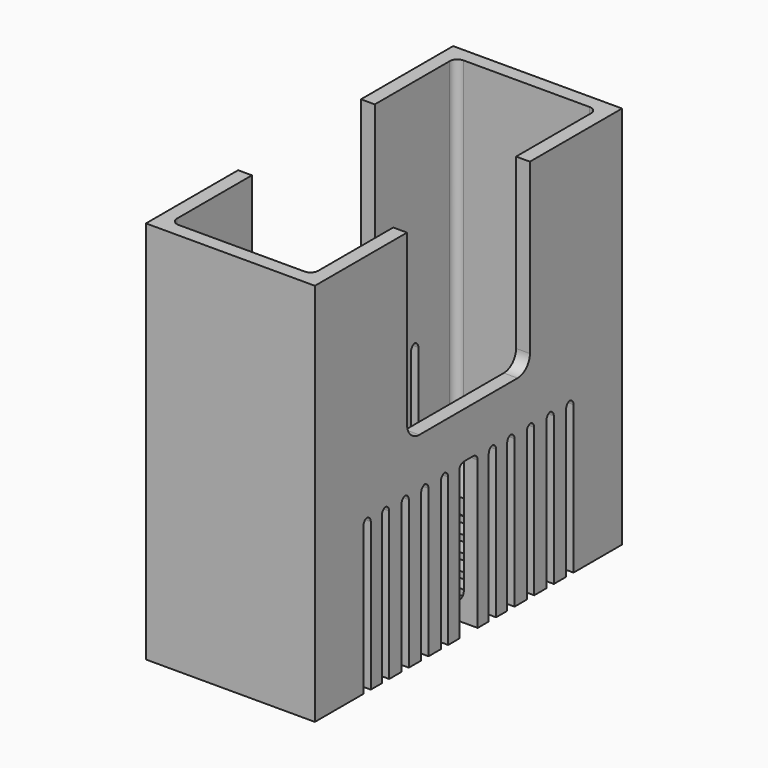
from build123d import *

# Parameters (mm, degrees)
F0_W            = 22
F0_H            = 50
F1_DEPTH        = 50
F2_T            = -1.8
F3_R            = 2
F4_W            = 33.5534993559
F4_H            = 3
F4_W_2          = 30.2066039294
F4_H_2          = 1.2
F4_W_3          = 26.0875225067
F4_W_4          = 25.4990821704
F4_W_5          = 26.8721096218
F4_W_6          = 25.5971541628
F4_W_7          = 23.243393749
F4_W_8          = 31.1466334388
F4_W_9          = 36.8653591722
F4_W_10         = 30.2834836766
F4_W_11         = 31.6123114899
F5_DEPTH        = 20
F6_W            = 20.4323772341
F6_H            = 6
F7_DEPTH        = 2
F8_W            = 20.5352026969
F8_H            = 6
F9_DEPTH        = 2
F10_R           = 1
F12_D           = 3.4
F12_CSINK_D     = 6.72
F12_CSINK_ANGLE = 90
F13_T1_DEPTH    = 1.8
F13_T3_DEPTH    = 1.8
F15_DEPTH       = 22.001


# Not quite as in the source:
# - a fillet or chamfer that OpenCascade refuses, or shapes differently, is made with other operations: its cross-section is extruded or revolved along the edge and cut away or added


with BuildPart() as f1:
    # F0 (on Top) → F1 (new body)
    with BuildSketch(Plane.XY):
        Rectangle(F0_W, F0_H)
    extrude(amount=F1_DEPTH)

    # F2
    f2_openings = [f1.faces().sort_by_distance(p)[0] for p in [
        (0, 0, 50),
    ]]
    offset(amount=F2_T, openings=f2_openings)

    # F3
    f3_edges = [f1.edges().sort_by_distance(p)[0] for p in [
        (9.2, 0, 1.8),
        (-9.2, 0, 1.8),
    ]]
    fillet(f3_edges, radius=F3_R)

    # F4 (on face) → F5 (cut)
    with BuildSketch(Plane(origin=(0, 0, 0), x_dir=(1, 0, 0), z_dir=(0, 0, -1))):
        with Locations((0.5022748373, 0)):
            Rectangle(F4_W, F4_H)
        with Locations((0.0301385298, 3.9)):
            Rectangle(F4_W_2, F4_H_2)
        with Locations((-0.4602279514, 10.3)):
            Rectangle(F4_W_3, F4_H_2)
        with Locations((-1.1467416771, -6.9)):
            Rectangle(F4_W_4, F4_H_2)
        with Locations((-0.6563747302, -10.1)):
            Rectangle(F4_W_5, F4_H_2)
        with Locations((-0.6073382683, -3.9)):
            Rectangle(F4_W_6, F4_H_2)
        with Locations((-0.2150442451, 7.1)):
            Rectangle(F4_W_7, F4_H_2)
        with Locations((0.075826887, 13.5)):
            Rectangle(F4_W_8, F4_H_2)
        with Locations((0.9949086234, -13.3)):
            Rectangle(F4_W_9, F4_H_2)
        with Locations((0.5074017681, 16.5)):
            Rectangle(F4_W_10, F4_H_2)
        with Locations((1.4125197195, -16.5)):
            Rectangle(F4_W_11, F4_H_2)
    extrude(amount=-F5_DEPTH, mode=Mode.SUBTRACT)

    # F6 (on face) → F7 (join)
    with BuildSketch(Plane.XY.offset(1.8)):
        with Locations((0.1267548651, 20.2)):
            Rectangle(F6_W, F6_H)
    extrude(amount=F7_DEPTH)

    # F8 (on face) → F9 (join)
    with BuildSketch(Plane.XY.offset(1.8)):
        with Locations((-0.0829612836, -20.2)):
            Rectangle(F8_W, F8_H)
    extrude(amount=F9_DEPTH)

    # F10
    f10_edges = [f1.edges().sort_by_distance(p)[0] for p in [
        (-9.2, -23.2, 26.9),
        (9.2, -23.2, 26.9),
        (9.2, 23.2, 26.9),
        (-9.2, 23.2, 26.9),
    ]]
    fillet(f10_edges, radius=F10_R)

    # F12 (through all)
    with Locations(Plane(origin=(0, 0, 0), x_dir=(1, 0, 0), z_dir=(0, 0, -1))):
        with Locations((0, 21), (0, -21)):
            CounterSinkHole(F12_D / 2, F12_CSINK_D / 2, counter_sink_angle=F12_CSINK_ANGLE)

    # F13: fillet of radius 0.75 on 44 edges, made by hand

    # F13_s2 → F13_t1 (join)
    with BuildSketch(Plane.YZ.offset(-11)):
        with BuildLine():
            ThreePointArc((-1.5, 19.25), (-1.2803300859, 19.7803300859), (-0.75, 20))
            Line((-0.75, 20), (-1.5, 20))
            Line((-1.5, 20), (-1.5, 19.25))
        make_face()
        with BuildLine():
            ThreePointArc((1.5, 19.25), (1.2803300859, 19.7803300859), (0.75, 20))
            Line((0.75, 20), (1.5, 20))
            Line((1.5, 20), (1.5, 19.25))
        make_face()
        with BuildLine():
            ThreePointArc((13.9, 19.25), (13.6803300859, 19.7803300859), (13.15, 20))
            Line((13.15, 20), (13.9, 20))
            Line((13.9, 20), (13.9, 19.25))
        make_face()
        with BuildLine():
            ThreePointArc((12.7, 19.25), (12.9196699141, 19.7803300859), (13.45, 20))
            Line((13.45, 20), (12.7, 20))
            Line((12.7, 20), (12.7, 19.25))
        make_face()
        with BuildLine():
            ThreePointArc((10.7, 19.25), (10.4803300859, 19.7803300859), (9.95, 20))
            Line((9.95, 20), (10.7, 20))
            Line((10.7, 20), (10.7, 19.25))
        make_face()
        with BuildLine():
            ThreePointArc((9.5, 19.25), (9.7196699141, 19.7803300859), (10.25, 20))
            Line((10.25, 20), (9.5, 20))
            Line((9.5, 20), (9.5, 19.25))
        make_face()
        with BuildLine():
            ThreePointArc((7.5, 19.25), (7.2803300859, 19.7803300859), (6.75, 20))
            Line((6.75, 20), (7.5, 20))
            Line((7.5, 20), (7.5, 19.25))
        make_face()
        with BuildLine():
            ThreePointArc((6.3, 19.25), (6.5196699141, 19.7803300859), (7.05, 20))
            Line((7.05, 20), (6.3, 20))
            Line((6.3, 20), (6.3, 19.25))
        make_face()
        with BuildLine():
            ThreePointArc((4.5, 19.25), (4.2803300859, 19.7803300859), (3.75, 20))
            Line((3.75, 20), (4.5, 20))
            Line((4.5, 20), (4.5, 19.25))
        make_face()
        with BuildLine():
            ThreePointArc((3.3, 19.25), (3.5196699141, 19.7803300859), (4.05, 20))
            Line((4.05, 20), (3.3, 20))
            Line((3.3, 20), (3.3, 19.25))
        make_face()
        with BuildLine():
            ThreePointArc((-3.3, 19.25), (-3.5196699141, 19.7803300859), (-4.05, 20))
            Line((-4.05, 20), (-3.3, 20))
            Line((-3.3, 20), (-3.3, 19.25))
        make_face()
        with BuildLine():
            ThreePointArc((-6.5, 19.25), (-6.7196699141, 19.7803300859), (-7.25, 20))
            Line((-7.25, 20), (-6.5, 20))
            Line((-6.5, 20), (-6.5, 19.25))
        make_face()
        with BuildLine():
            ThreePointArc((-9.7, 19.25), (-9.9196699141, 19.7803300859), (-10.45, 20))
            Line((-10.45, 20), (-9.7, 20))
            Line((-9.7, 20), (-9.7, 19.25))
        make_face()
        with BuildLine():
            ThreePointArc((-12.9, 19.25), (-13.1196699141, 19.7803300859), (-13.65, 20))
            Line((-13.65, 20), (-12.9, 20))
            Line((-12.9, 20), (-12.9, 19.25))
        make_face()
        with BuildLine():
            ThreePointArc((-14.1, 19.25), (-13.8803300859, 19.7803300859), (-13.35, 20))
            Line((-13.35, 20), (-14.1, 20))
            Line((-14.1, 20), (-14.1, 19.25))
        make_face()
        with BuildLine():
            ThreePointArc((-10.9, 19.25), (-10.6803300859, 19.7803300859), (-10.15, 20))
            Line((-10.15, 20), (-10.9, 20))
            Line((-10.9, 20), (-10.9, 19.25))
        make_face()
        with BuildLine():
            ThreePointArc((-7.7, 19.25), (-7.4803300859, 19.7803300859), (-6.95, 20))
            Line((-6.95, 20), (-7.7, 20))
            Line((-7.7, 20), (-7.7, 19.25))
        make_face()
        with BuildLine():
            ThreePointArc((-4.5, 19.25), (-4.2803300859, 19.7803300859), (-3.75, 20))
            Line((-3.75, 20), (-4.5, 20))
            Line((-4.5, 20), (-4.5, 19.25))
        make_face()
        with BuildLine():
            ThreePointArc((15.9, 19.25), (16.1196699141, 19.7803300859), (16.65, 20))
            Line((16.65, 20), (15.9, 20))
            Line((15.9, 20), (15.9, 19.25))
        make_face()
        with BuildLine():
            ThreePointArc((17.1, 19.25), (16.8803300859, 19.7803300859), (16.35, 20))
            Line((16.35, 20), (17.1, 20))
            Line((17.1, 20), (17.1, 19.25))
        make_face()
        with BuildLine():
            ThreePointArc((-17.1, 19.25), (-16.8803300859, 19.7803300859), (-16.35, 20))
            Line((-16.35, 20), (-17.1, 20))
            Line((-17.1, 20), (-17.1, 19.25))
        make_face()
        with BuildLine():
            ThreePointArc((-15.9, 19.25), (-16.1196699141, 19.7803300859), (-16.65, 20))
            Line((-16.65, 20), (-15.9, 20))
            Line((-15.9, 20), (-15.9, 19.25))
        make_face()
    extrude(amount=F13_T1_DEPTH)

    # F13_s4 → F13_t3 (join)
    with BuildSketch(Plane.YZ.offset(9.2)):
        with BuildLine():
            ThreePointArc((1.5, 19.25), (1.2803300859, 19.7803300859), (0.75, 20))
            Line((0.75, 20), (1.5, 20))
            Line((1.5, 20), (1.5, 19.25))
        make_face()
        with BuildLine():
            ThreePointArc((-1.5, 19.25), (-1.2803300859, 19.7803300859), (-0.75, 20))
            Line((-0.75, 20), (-1.5, 20))
            Line((-1.5, 20), (-1.5, 19.25))
        make_face()
        with BuildLine():
            ThreePointArc((-13.65, 20), (-13.1196699141, 19.7803300859), (-12.9, 19.25))
            Line((-12.9, 19.25), (-12.9, 20))
            Line((-12.9, 20), (-13.65, 20))
        make_face()
        with BuildLine():
            ThreePointArc((-10.45, 20), (-9.9196699141, 19.7803300859), (-9.7, 19.25))
            Line((-9.7, 19.25), (-9.7, 20))
            Line((-9.7, 20), (-10.45, 20))
        make_face()
        with BuildLine():
            ThreePointArc((-7.25, 20), (-6.7196699141, 19.7803300859), (-6.5, 19.25))
            Line((-6.5, 19.25), (-6.5, 20))
            Line((-6.5, 20), (-7.25, 20))
        make_face()
        with BuildLine():
            ThreePointArc((-4.05, 20), (-3.5196699141, 19.7803300859), (-3.3, 19.25))
            Line((-3.3, 19.25), (-3.3, 20))
            Line((-3.3, 20), (-4.05, 20))
        make_face()
        with BuildLine():
            ThreePointArc((4.5, 19.25), (4.2803300859, 19.7803300859), (3.75, 20))
            Line((3.75, 20), (4.5, 20))
            Line((4.5, 20), (4.5, 19.25))
        make_face()
        with BuildLine():
            ThreePointArc((7.5, 19.25), (7.2803300859, 19.7803300859), (6.75, 20))
            Line((6.75, 20), (7.5, 20))
            Line((7.5, 20), (7.5, 19.25))
        make_face()
        with BuildLine():
            ThreePointArc((10.7, 19.25), (10.4803300859, 19.7803300859), (9.95, 20))
            Line((9.95, 20), (10.7, 20))
            Line((10.7, 20), (10.7, 19.25))
        make_face()
        with BuildLine():
            ThreePointArc((13.9, 19.25), (13.6803300859, 19.7803300859), (13.15, 20))
            Line((13.15, 20), (13.9, 20))
            Line((13.9, 20), (13.9, 19.25))
        make_face()
        with BuildLine():
            ThreePointArc((-14.1, 19.25), (-13.8803300859, 19.7803300859), (-13.35, 20))
            Line((-13.35, 20), (-14.1, 20))
            Line((-14.1, 20), (-14.1, 19.25))
        make_face()
        with BuildLine():
            ThreePointArc((-10.9, 19.25), (-10.6803300859, 19.7803300859), (-10.15, 20))
            Line((-10.15, 20), (-10.9, 20))
            Line((-10.9, 20), (-10.9, 19.25))
        make_face()
        with BuildLine():
            ThreePointArc((-7.7, 19.25), (-7.4803300859, 19.7803300859), (-6.95, 20))
            Line((-6.95, 20), (-7.7, 20))
            Line((-7.7, 20), (-7.7, 19.25))
        make_face()
        with BuildLine():
            ThreePointArc((-4.5, 19.25), (-4.2803300859, 19.7803300859), (-3.75, 20))
            Line((-3.75, 20), (-4.5, 20))
            Line((-4.5, 20), (-4.5, 19.25))
        make_face()
        with BuildLine():
            ThreePointArc((4.05, 20), (3.5196699141, 19.7803300859), (3.3, 19.25))
            Line((3.3, 19.25), (3.3, 20))
            Line((3.3, 20), (4.05, 20))
        make_face()
        with BuildLine():
            ThreePointArc((7.05, 20), (6.5196699141, 19.7803300859), (6.3, 19.25))
            Line((6.3, 19.25), (6.3, 20))
            Line((6.3, 20), (7.05, 20))
        make_face()
        with BuildLine():
            ThreePointArc((10.25, 20), (9.7196699141, 19.7803300859), (9.5, 19.25))
            Line((9.5, 19.25), (9.5, 20))
            Line((9.5, 20), (10.25, 20))
        make_face()
        with BuildLine():
            ThreePointArc((13.45, 20), (12.9196699141, 19.7803300859), (12.7, 19.25))
            Line((12.7, 19.25), (12.7, 20))
            Line((12.7, 20), (13.45, 20))
        make_face()
        with BuildLine():
            ThreePointArc((-17.1, 19.25), (-16.8803300859, 19.7803300859), (-16.35, 20))
            Line((-16.35, 20), (-17.1, 20))
            Line((-17.1, 20), (-17.1, 19.25))
        make_face()
        with BuildLine():
            ThreePointArc((-16.65, 20), (-16.1196699141, 19.7803300859), (-15.9, 19.25))
            Line((-15.9, 19.25), (-15.9, 20))
            Line((-15.9, 20), (-16.65, 20))
        make_face()
        with BuildLine():
            ThreePointArc((17.1, 19.25), (16.8803300859, 19.7803300859), (16.35, 20))
            Line((16.35, 20), (17.1, 20))
            Line((17.1, 20), (17.1, 19.25))
        make_face()
        with BuildLine():
            ThreePointArc((16.65, 20), (16.1196699141, 19.7803300859), (15.9, 19.25))
            Line((15.9, 19.25), (15.9, 20))
            Line((15.9, 20), (16.65, 20))
        make_face()
    extrude(amount=F13_T3_DEPTH)

    # F14 (on face) → F15 (cut, through all)
    with BuildSketch(Plane.YZ.offset(11)):
        with BuildLine():
            Line((10, 50), (-10, 50))
            Line((-10, 50), (-10, 28))
            ThreePointArc((-10, 28), (-9.4142135624, 26.5857864376), (-8, 26))
            Line((-8, 26), (8, 26))
            ThreePointArc((8, 26), (9.4142135624, 26.5857864376), (10, 28))
            Line((10, 28), (10, 50))
        make_face()
    extrude(amount=-F15_DEPTH, mode=Mode.SUBTRACT)


solid = f1.part
